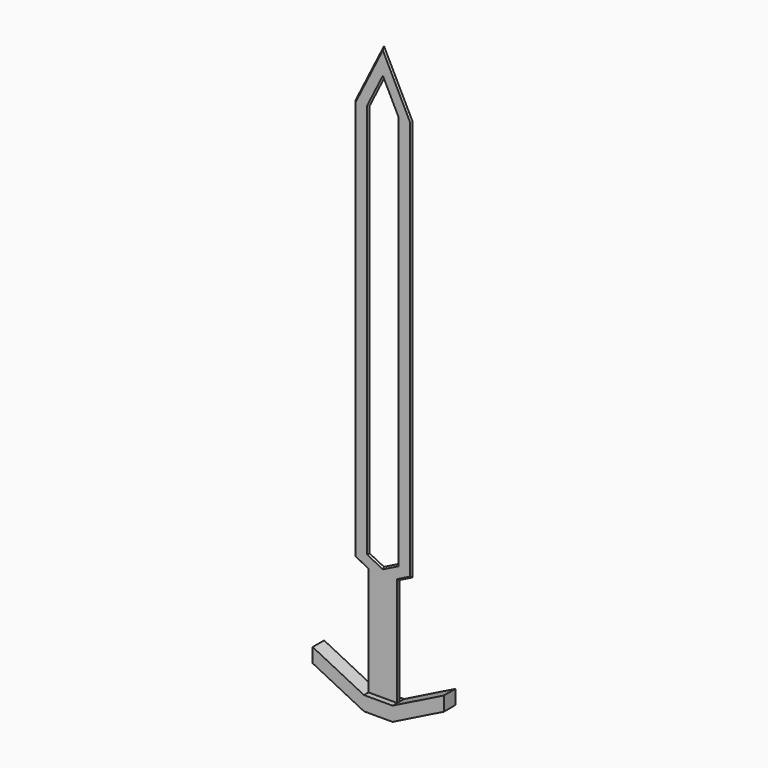
from build123d import *

# Parameters (mm, degrees)
F1_DEPTH = 0.635
F2_SIZE  = 0.63499
F3_DEPTH = 3.175
F4_SIZE  = 0.63499


# Not quite as in the source:
# - a fillet or chamfer is up to 0.001 mm smaller than in the source, because OpenCascade refuses the exact size


with BuildPart() as f1:
    # F0 (on Front) → F1 (new body, symmetric)
    with BuildSketch(Plane.XZ):
        Polygon((12.7, 177.8), (0, 203.2), (-12.7, 177.8), (-12.7, 0), (-6.35, -3.175), (-6.35, -50.8), (0, -50.8), (6.35, -50.8), (6.35, -3.175), (12.7, 0), align=None)
        Polygon((-6.35, 177.8), (0, 190.5), (6.35, 177.8), (6.35, 3.175), (0, 0), (-6.35, 3.175), align=None, mode=Mode.SUBTRACT)
    extrude(amount=F1_DEPTH, both=True)

    # F2 (size 0.635 in the source; OpenCascade refuses exactly that, so slightly less here)
    f2_edges = [f1.edges().sort_by_distance(p)[0] for p in [
        (12.7, -0.635, 88.9),
        (6.35, -0.635, 190.5),
        (-6.35, -0.635, 190.5),
        (-12.7, -0.635, 88.9),
        (-9.525, -0.635, -1.5875),
        (9.525, -0.635, -1.5875),
        (-9.525, 0.635, -1.5875),
        (9.525, 0.635, -1.5875),
        (-12.7, 0.635, 88.9),
        (12.7, 0.635, 88.9),
        (-6.35, 0.635, 190.5),
        (6.35, 0.635, 190.5),
    ]]
    chamfer(f2_edges, length=F2_SIZE)

    # F0 (on Front) → F3 (join, symmetric)
    with BuildSketch(Plane.XZ):
        Polygon((0, -50.8), (-6.35, -50.8), (-29.0684506514, -39.4407746743), (-29.0684506514, -45.7907746743), (-6.35, -57.15), (-3.175, -57.15), (0, -57.15), (3.175, -57.15), (6.35, -57.15), (29.0684506514, -45.7907746743), (29.0684506514, -39.4407746743), (6.35, -50.8), align=None)
    extrude(amount=F3_DEPTH, both=True)

    # F4 (size 0.635 in the source; OpenCascade refuses exactly that, so slightly less here)
    f4_edges = [f1.edges().sort_by_distance(p)[0] for p in [
        (6.35, -0.635, 90.4875),
        (-6.35, -0.635, 90.4875),
        (3.175, -0.635, 1.5875),
        (-3.175, -0.635, 1.5875),
        (-3.175, -0.635, 184.15),
        (3.175, -0.635, 184.15),
        (3.175, 0.635, 184.15),
        (-3.175, 0.635, 184.15),
        (-6.35, 0.635, 90.4875),
        (6.35, 0.635, 90.4875),
        (-3.175, 0.635, 1.5875),
        (3.175, 0.635, 1.5875),
    ]]
    chamfer(f4_edges, length=F4_SIZE)


solid = f1.part
